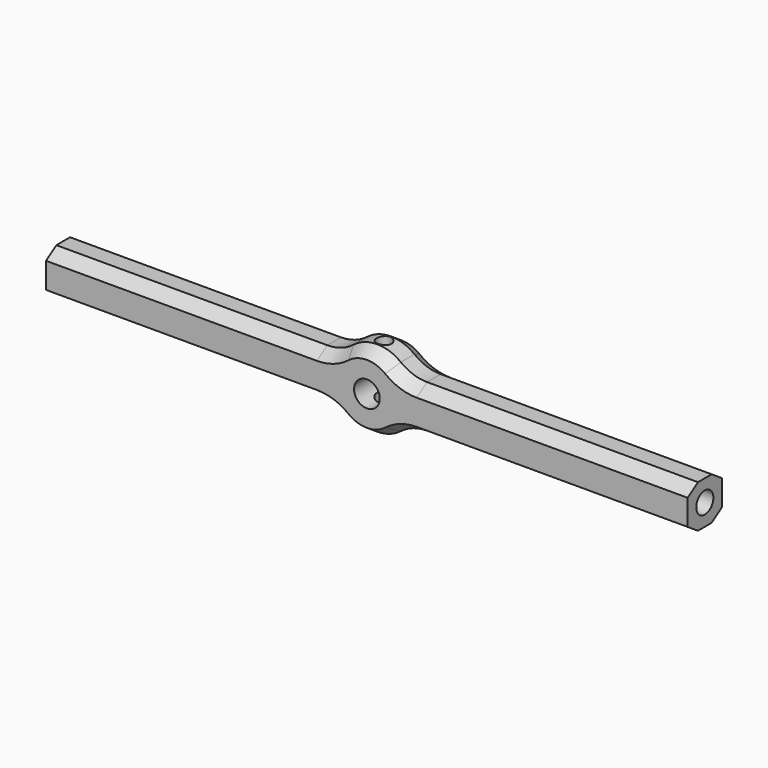
from build123d import *

# Parameters (mm, degrees)
F0_R          = 3
F1_DEPTH      = 10
F2_R          = 2.5
F3_DEPTH      = 25
F4_R          = 1.75
F5_DEPTH      = 9.001
F5_DEPTH_BACK = 9.001
F6_R          = 10
F7_SIZE2      = 3
F7_SIZE       = 2
F7_2_SIZE2    = 3
F7_2_SIZE     = 2


# Not quite as in the source:
# - a pattern or mirror of a feature is missing from the dataset's text; its kind, count and spacing are read off the source's solid


with BuildPart() as f1:
    # F0 (on Front) → F1 (new body)
    with BuildSketch(Plane.XZ):
        with BuildLine():
            Line((75, 5), (7.4833147735, 5))
            ThreePointArc((7.4833147735, 5), (0, 9), (-7.4833147735, 5))
            Line((-7.4833147735, 5), (-75, 5))
            Line((-75, 5), (-75, -5))
            Line((-75, -5), (-7.4833147735, -5))
            ThreePointArc((-7.4833147735, -5), (0, -9), (7.4833147735, -5))
            Line((7.4833147735, -5), (75, -5))
            Line((75, -5), (75, 5))
        make_face()
        Circle(F0_R, mode=Mode.SUBTRACT)
    extrude(amount=F1_DEPTH)

    # F2 (on face) → F3 (cut)
    with BuildSketch(Plane(origin=(-75, 0, 0), x_dir=(0, -1, 0), z_dir=(-1, 0, 0))):
        with Locations((5, 0)):
            Circle(F2_R)
    f3 = extrude(amount=-F3_DEPTH, mode=Mode.SUBTRACT)

    # F3_copies: F3 across plane
    add(f3.mirror(Plane(origin=(0, 0, 0), x_dir=(0, 0, 1), z_dir=(1, 0, 0))), mode=Mode.SUBTRACT)

    # F4 (on Top) → F5 (cut, two sides)
    with BuildSketch(Plane.XY) as f5_sk:
        with Locations((0, -5)):
            Circle(F4_R)
    extrude(amount=-F5_DEPTH, mode=Mode.SUBTRACT)
    extrude(f5_sk.sketch, amount=F5_DEPTH_BACK, mode=Mode.SUBTRACT)

    # F6
    f6_edges = [f1.edges().sort_by_distance(p)[0] for p in [
        (-7.483315, -5, 5),
        (7.483315, -5, 5),
        (7.483315, -5, -5),
        (-7.483315, -5, -5),
    ]]
    fillet(f6_edges, radius=F6_R)

    # F7
    f7_edges = [f1.edges().sort_by_distance(p)[0] for p in [
        (-43.330952, -10, 5),
        (-43.330952, -10, -5),
    ]]
    f7_side = f1.faces().sort_by_distance((43.330952, -10, -3.489239))[0]
    chamfer(f7_edges, length=F7_SIZE, length2=F7_SIZE2, reference=f7_side)

    # F7#2
    f7_2_edges = [f1.edges().sort_by_distance(p)[0] for p in [
        (-43.330952, 0, 5),
        (-43.330952, 0, -5),
    ]]
    f7_2_side = f1.faces().sort_by_distance((43.330952, 0, -3.489239))[0]
    chamfer(f7_2_edges, length=F7_2_SIZE, length2=F7_2_SIZE2, reference=f7_2_side)


solid = f1.part
